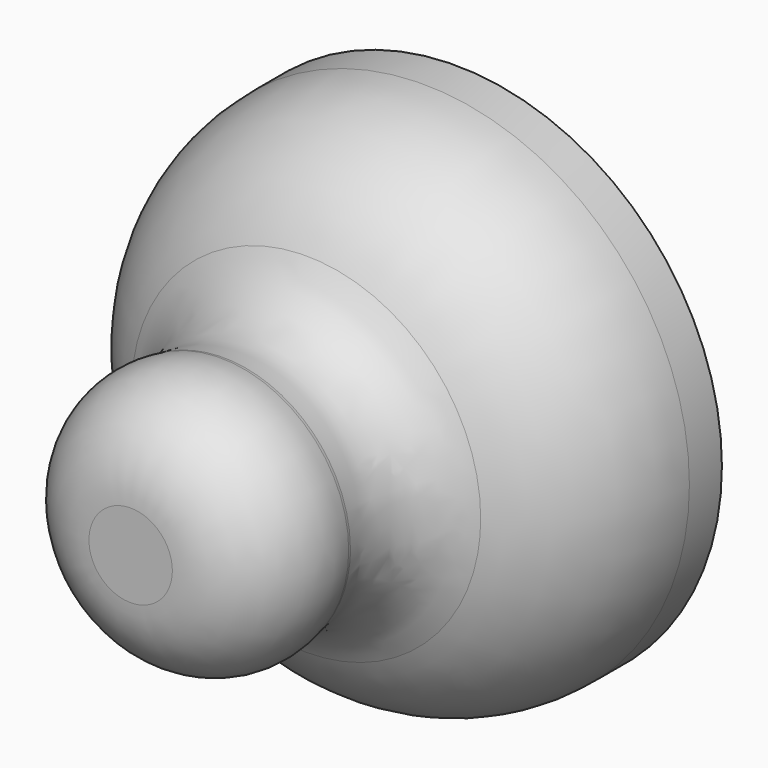
from build123d import *

# Parameters (mm, degrees)
F0_R      = 32.7709743637
F1_DEPTH  = 25
F2_R      = 20
F1_FACE_R = 12.7709743637
F3_DEPTH  = 25
F3_TAPER  = -15
F4_R      = 11


with BuildPart() as f1:
    # F0 (on Front) → F1 (new body)
    with BuildSketch(Plane.XZ):
        Circle(F0_R)
    extrude(amount=F1_DEPTH)

    # F2
    f2_edges = [f1.edges().sort_by_distance(p)[0] for p in [
        (-32.770974, -25, 0),
    ]]
    fillet(f2_edges, radius=F2_R)

    # F1_face (on face) → F3 (join)
    with BuildSketch(Plane.XZ.offset(25)):
        Circle(F1_FACE_R)
    extrude(amount=F3_DEPTH, taper=F3_TAPER)

    # F4
    f4_edges = [f1.edges().sort_by_distance(p)[0] for p in [
        (-19.469704, -50, 0),
        (-12.770974, -25, 0),
    ]]
    fillet(f4_edges, radius=F4_R)


solid = f1.part
